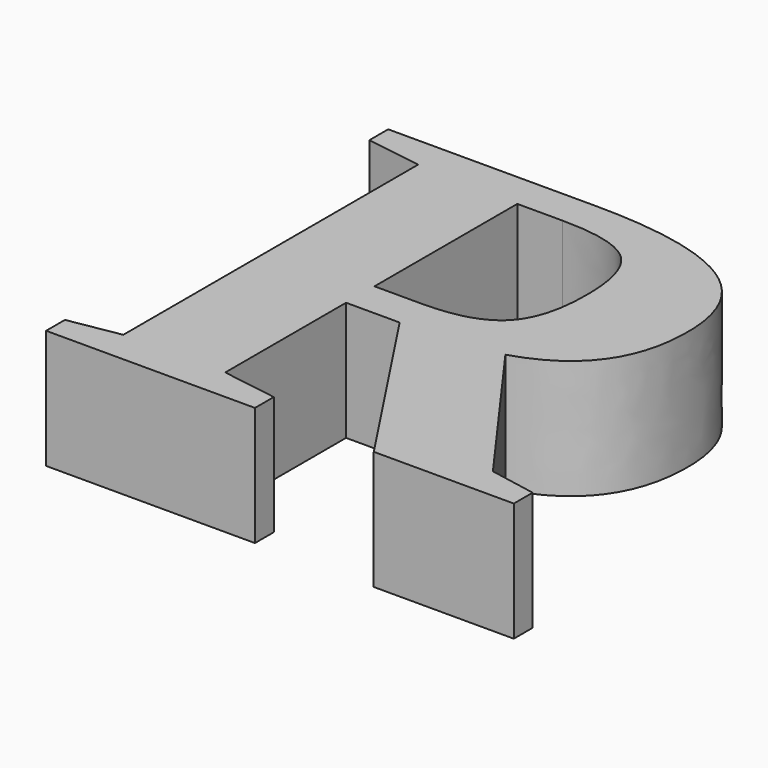
from build123d import *

# Parameters (mm, degrees)
F0_TEXT_SIZE = 141.1111111111
F1_DEPTH     = 25.4


# Not quite as in the source:
# - Text() gives the source's letters only with a copy of the font that has no kerning and outlines rounded to 1/6400 em; it was checked with that copy


with BuildPart() as f1:
    # F0 (on Top) → F1 (new body)
    with BuildSketch(Plane.XY):
        with Locations((-27.6588893265, -68.2137652326)):
            Text('R', F0_TEXT_SIZE, font='Tinos', font_style=FontStyle.BOLD, text_align=(TextAlign.LEFT, TextAlign.BOTTOM))
    extrude(amount=F1_DEPTH)


solid = f1.part
